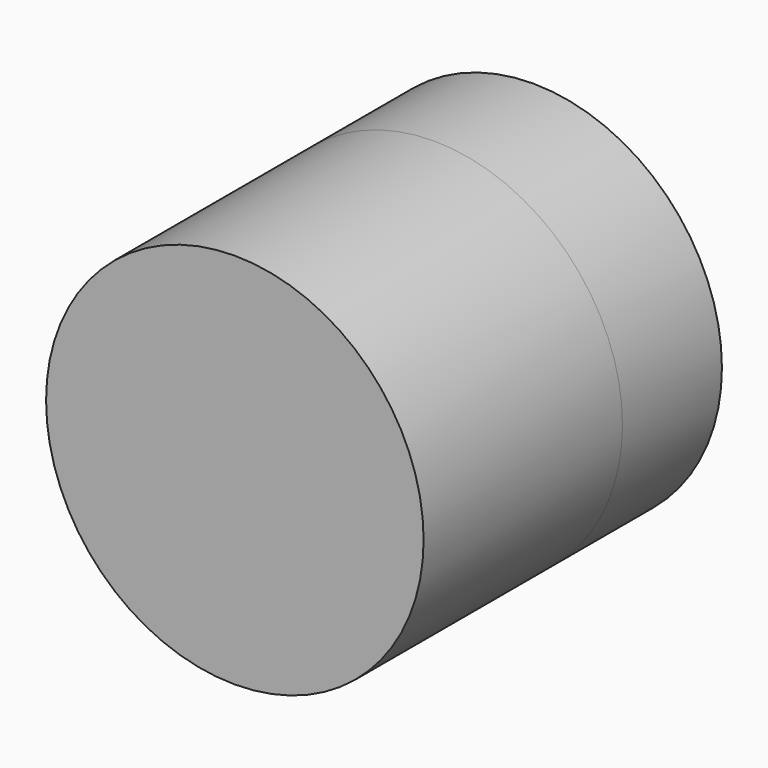
from build123d import *

# Parameters (mm, degrees)
F0_R     = 38.572234299
F1_DEPTH = 25.4
F2_DEPTH = 25.4
F3_DEPTH = 25.4


with BuildPart() as f1:
    # F0 (on Front) → F1 (new body)
    with BuildSketch(Plane.XZ):
        with Locations((-53.8619197905, 27.4006854743)):
            Circle(F0_R)
    extrude(amount=F1_DEPTH)

    # F2 (add): faces of the model
    f2_faces = [f1.faces().sort_by_distance(p)[0] for p in [
        (-53.8619197905, -25.4, 27.4006854743),
        (-53.8619197905, 0, 27.4006854743),
    ]]
    extrude(f2_faces, amount=F2_DEPTH, dir=(0, -1, 0))

    # F3 (add): a face of the model
    f3_faces = [f1.faces().sort_by_distance(p)[0] for p in [
        (-53.8619197905, 0, 27.4006854743),
    ]]
    extrude(f3_faces, amount=F3_DEPTH)


solid = f1.part
